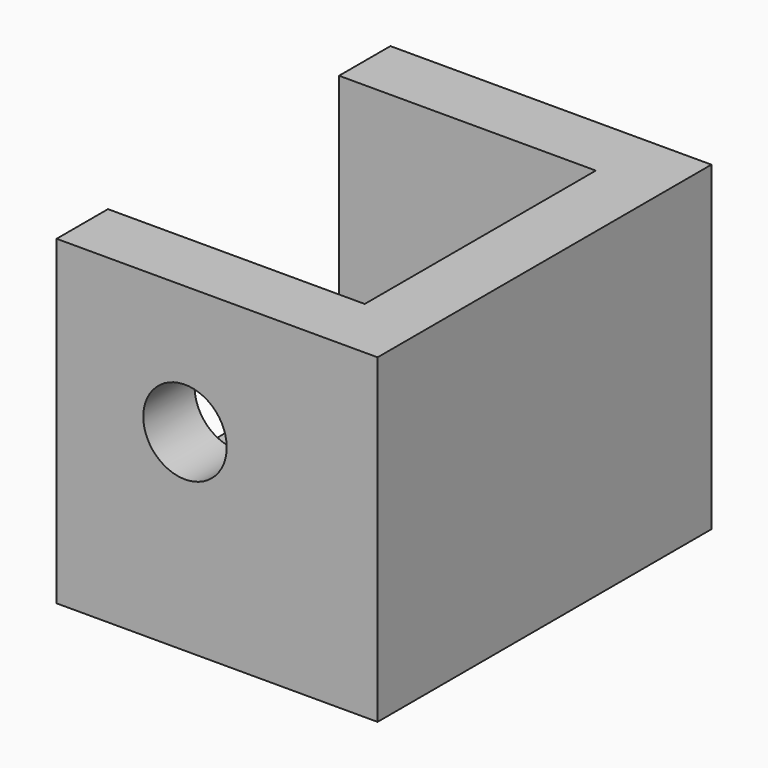
from build123d import *

# Parameters (mm, degrees)
F1_DEPTH = 10
F2_W     = 9
F2_H     = 2
F3_DEPTH = 8
F4_R     = 1.3
F5_DEPTH = 2


# Not quite as in the source:
# - a feature names something its author has since deleted; it is built from what else it names


with BuildPart() as f1:
    # F0 (on Top) → F1 (new body)
    with BuildSketch(Plane.XY):
        Polygon((-5, -6.5), (5, -6.5), (5, 6.5), (-5, 6.5), (-5, 4.5), (-3, 4.5), (3, 4.5), (3, -4.5), (-3, -4.5), (-5, -4.5), align=None)
    extrude(amount=F1_DEPTH)

    # F2 (on face) → F3 (join)
    with BuildSketch(Plane(origin=(3, 0, 0), x_dir=(0, -1, 0), z_dir=(-1, 0, 0))):
        with Locations((0, 1)):
            Rectangle(F2_W, F2_H)
    extrude(amount=F3_DEPTH)

    # F4 (on face) → F5 (cut, through all)
    with BuildSketch(Plane.XZ.offset(6.5)):
        with Locations((-1, 6)):
            Circle(F4_R)
    extrude(amount=-F5_DEPTH, mode=Mode.SUBTRACT)


solid = f1.part
